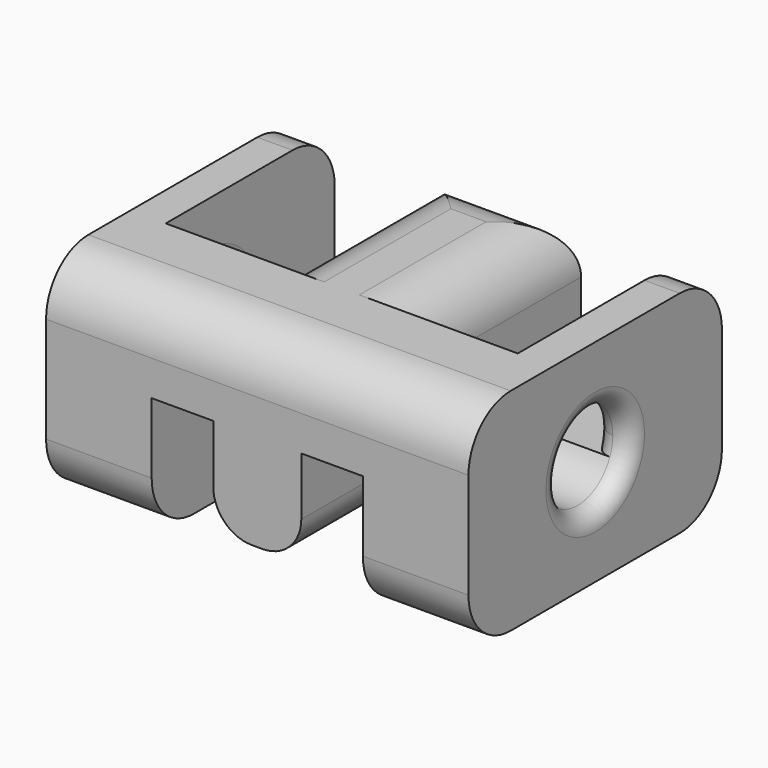
from build123d import *

# Parameters (mm, degrees)
F0_W          = 12
F0_H          = 9
F1_DEPTH      = 6
F2_W          = 3
F2_H          = 6
F3_DEPTH      = 3.5
F4_W          = 6
F4_H          = 6.5
F5_DEPTH      = 3.5
F6_R          = 1.25
F7_DEPTH      = 3
F8_R          = 1.25
F9_DEPTH      = 3.001
F10_R         = 1.5
F11_W         = 2.5
F11_H         = 6.5
F12_DEPTH     = 2.75
F13_R         = 1.1
F14_T8_ANGLE  = 247.5355258221
F14_T13_ANGLE = 80.8755372564
F14_T18_ANGLE = 260.9918579461
F14_T24_ANGLE = 247.5355258221
F14_T29_ANGLE = 260.9918579461
F14_T35_ANGLE = 80.8755372564


# Not quite as in the source:
# - a fillet or chamfer that OpenCascade refuses, or shapes differently, is made with other operations: its cross-section is extruded or revolved along the edge and cut away or added


with BuildPart() as f1:
    # F0 (on Top) → F1 (new body)
    with BuildSketch(Plane.XY):
        Rectangle(F0_W, F0_H)
    extrude(amount=F1_DEPTH)

    # F2 (on face) → F3 (cut)
    with BuildSketch(Plane.XY.offset(6)):
        with Locations((3.5, 1.5)):
            Rectangle(F2_W, F2_H)
        with Locations((-3.5, 1.5)):
            Rectangle(F2_W, F2_H)
    extrude(amount=-F3_DEPTH, mode=Mode.SUBTRACT)

    # F4 (on face) → F5 (cut)
    with BuildSketch(Plane(origin=(0, 0, 0), x_dir=(1, 0, 0), z_dir=(0, 0, -1))):
        with Locations((0, 1.25)):
            Rectangle(F4_W, F4_H)
    extrude(amount=-F5_DEPTH, mode=Mode.SUBTRACT)

    # F6 (on face) → F7 (cut)
    with BuildSketch(Plane.YZ.offset(6)):
        with Locations((0, 3)):
            Circle(F6_R)
    extrude(amount=-F7_DEPTH, mode=Mode.SUBTRACT)

    # F8 (on face) → F9 (cut, through all)
    with BuildSketch(Plane(origin=(-6, 0, 0), x_dir=(0, -1, 0), z_dir=(-1, 0, 0))):
        with Locations((0, 3)):
            Circle(F8_R)
    extrude(amount=-F9_DEPTH, mode=Mode.SUBTRACT)

    # F10
    f10_edges = [f1.edges().sort_by_distance(p)[0] for p in [
        (2, 1.5, 6),
        (-2, 1.5, 6),
        (0, -4.5, 6),
        (-4.5, -4.5, 0),
        (4.5, -4.5, 0),
        (0, 4.5, 0),
        (-5.5, 4.5, 6),
        (5.5, 4.5, 6),
        (0, 4.5, 6),
    ]]
    fillet(f10_edges, radius=F10_R)

    # F11 (on face) → F12 (join)
    with BuildSketch(Plane(origin=(0, 0, 3.5), x_dir=(1, 0, 0), z_dir=(0, 0, -1))):
        with Locations((0, 1.25)):
            Rectangle(F11_W, F11_H)
    extrude(amount=F12_DEPTH)

    # F13
    f13_edges = [f1.edges().sort_by_distance(p)[0] for p in [
        (-1.25, -1.25, 0.75),
        (1.25, -1.25, 0.75),
    ]]
    fillet(f13_edges, radius=F13_R)

    # F14: fillet of radius 0.5 on 7 edges, made by hand

    # F14_s1 → F14_t2 (revolve, cut)
    with BuildSketch(Plane.XY.offset(3)):
        with BuildLine():
            ThreePointArc((6, 1.75), (5.8535533906, 1.3964466094), (5.5, 1.25))
            Line((5.5, 1.25), (6, 1.25))
            Line((6, 1.25), (6, 1.75))
        make_face()
    revolve(axis=Axis((6, 0, 3), (1, 0, 0)), mode=Mode.SUBTRACT)

    # F14_s3 → F14_t4 (revolve, cut)
    with BuildSketch(Plane.XY.offset(3)):
        with BuildLine():
            ThreePointArc((-6, -1.75), (-5.8535533906, -1.3964466094), (-5.5, -1.25))
            Line((-5.5, -1.25), (-6, -1.25))
            Line((-6, -1.25), (-6, -1.75))
        make_face()
    revolve(axis=Axis((-6, 0, 3), (-1, 0, 0)), mode=Mode.SUBTRACT)


with BuildPart() as f14_tool6:
    # F14_s7 → F14_t8 (revolve)
    with BuildSketch(Plane(origin=(0, -1.3861749524, 2.0731657713), x_dir=(1, 0, 0), z_dir=(0, -0.5558279796, 0.8312973338))):
        with BuildLine():
            ThreePointArc((-3, 3.4174839388), (-3.1464466094, 3.0639305482), (-3.5, 2.9174839388))
            Line((-3.5, 2.9174839388), (-3, 2.9174839388))
            Line((-3, 2.9174839388), (-3, 3.4174839388))
        make_face()
    revolve(axis=Axis((-3, 0, 3), (-1, 0, 0)), revolution_arc=F14_T8_ANGLE)

    split(bisect_by=Plane.XY.offset(3.5), keep=Keep.BOTTOM)


with BuildPart() as f1_1:
    add(f1.part)

    # F14_t5: cut F14_tool6
    add(f14_tool6.part, mode=Mode.SUBTRACT)


with BuildPart() as f14_tool11:
    # F14_s12 → F14_t13 (revolve)
    with BuildSketch(Plane(origin=(0, 0.469718994, 0.0754425014), x_dir=(1, 0, 0), z_dir=(0, -0.9873461903, -0.1585796345))):
        with BuildLine():
            ThreePointArc((5.5, 1.7120385709), (5.1464466094, 1.5655919615), (5, 1.2120385709))
            Line((5, 1.2120385709), (5, 1.7120385709))
            Line((5, 1.7120385709), (5.5, 1.7120385709))
        make_face()
    revolve(axis=Axis((5, 0, 3), (1, 0, 0)), revolution_arc=F14_T13_ANGLE)

    split(bisect_by=Plane.XY.offset(2.5), keep=Keep.TOP)


with BuildPart() as f1_2:
    add(f1_1.part)

    # F14_t10: cut F14_tool11
    add(f14_tool11.part, mode=Mode.SUBTRACT)


with BuildPart() as f14_tool16:
    # F14_s17 → F14_t18 (revolve)
    with BuildSketch(Plane.XY.offset(3)):
        with BuildLine():
            ThreePointArc((5.5, 1.25), (5.1464466094, 1.3964466094), (5, 1.75))
            Line((5, 1.75), (5, 1.25))
            Line((5, 1.25), (5.5, 1.25))
        make_face()
    revolve(axis=Axis((5, 0, 3), (1, 0, 0)), revolution_arc=F14_T18_ANGLE)

    split(bisect_by=Plane.XZ.offset(1.5), keep=Keep.BOTTOM)

    split(bisect_by=Plane.XY.offset(2.5), keep=Keep.TOP)


with BuildPart() as f1_3:
    add(f1_2.part)

    # F14_t15: cut F14_tool16
    add(f14_tool16.part, mode=Mode.SUBTRACT)


with BuildPart() as f14_tool22:
    # F14_s23 → F14_t24 (revolve)
    with BuildSketch(Plane(origin=(0, 1.3861749524, 2.0731657713), x_dir=(1, 0, 0), z_dir=(0, 0.5558279796, 0.8312973338))):
        with BuildLine():
            ThreePointArc((3, -3.4174839388), (3.1464466094, -3.0639305482), (3.5, -2.9174839388))
            Line((3.5, -2.9174839388), (3, -2.9174839388))
            Line((3, -2.9174839388), (3, -3.4174839388))
        make_face()
    revolve(axis=Axis((3, 0, 3), (1, 0, 0)), revolution_arc=F14_T24_ANGLE)

    split(bisect_by=Plane.XY.offset(3.5), keep=Keep.BOTTOM)


with BuildPart() as f1_4:
    add(f1_3.part)

    # F14_t21: cut F14_tool22
    add(f14_tool22.part, mode=Mode.SUBTRACT)


with BuildPart() as f14_tool27:
    # F14_s28 → F14_t29 (revolve)
    with BuildSketch(Plane.XY.offset(3)):
        with BuildLine():
            ThreePointArc((-5.5, -1.25), (-5.1464466094, -1.3964466094), (-5, -1.75))
            Line((-5, -1.75), (-5, -1.25))
            Line((-5, -1.25), (-5.5, -1.25))
        make_face()
    revolve(axis=Axis((-5, 0, 3), (-1, 0, 0)), revolution_arc=F14_T29_ANGLE)

    split(bisect_by=Plane.XZ.offset(1.5), keep=Keep.BOTTOM)

    split(bisect_by=Plane.XY.offset(2.5), keep=Keep.TOP)


with BuildPart() as f1_5:
    add(f1_4.part)

    # F14_t26: cut F14_tool27
    add(f14_tool27.part, mode=Mode.SUBTRACT)


with BuildPart() as f14_tool33:
    # F14_s34 → F14_t35 (revolve)
    with BuildSketch(Plane(origin=(0, -0.469718994, 0.0754425014), x_dir=(1, 0, 0), z_dir=(0, 0.9873461903, -0.1585796345))):
        with BuildLine():
            ThreePointArc((-5.5, -1.7120385709), (-5.1464466094, -1.5655919615), (-5, -1.2120385709))
            Line((-5, -1.2120385709), (-5, -1.7120385709))
            Line((-5, -1.7120385709), (-5.5, -1.7120385709))
        make_face()
    revolve(axis=Axis((-5, 0, 3), (-1, 0, 0)), revolution_arc=F14_T35_ANGLE)

    split(bisect_by=Plane.XZ.offset(1.5), keep=Keep.BOTTOM)

    split(bisect_by=Plane.XY.offset(2.5), keep=Keep.TOP)


with BuildPart() as f1_6:
    add(f1_5.part)

    # F14_t32: cut F14_tool33
    add(f14_tool33.part, mode=Mode.SUBTRACT)


solid = f1_6.part
